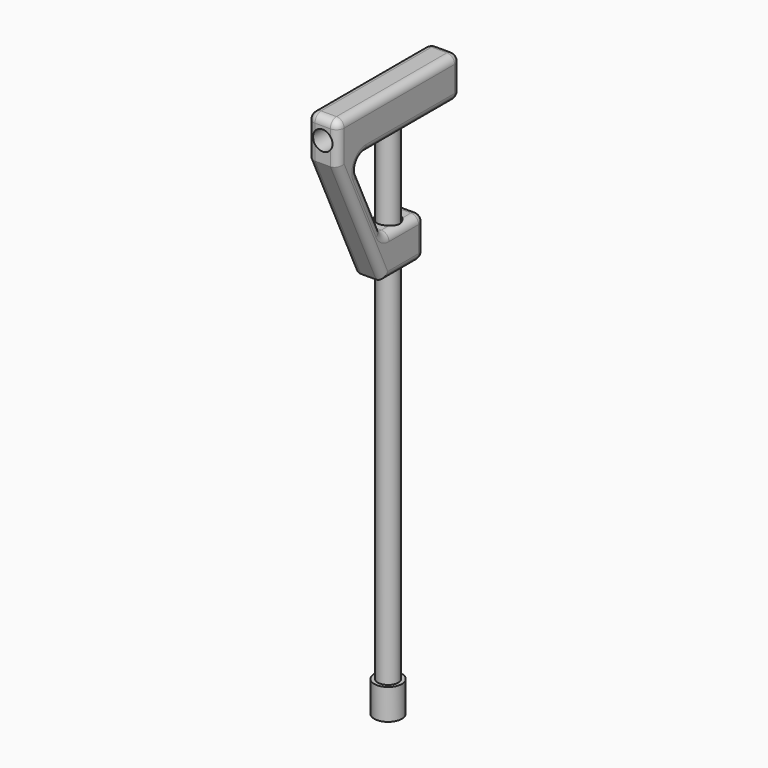
from build123d import *

# Parameters (mm, degrees)
F0_R          = 1.35
F1_DEPTH      = 3
F2_R          = 1
F3_DEPTH      = 50
F4_W          = 5
F4_H          = 4
F5_DEPTH      = 1.5
F6_R          = 1.1
F7_DEPTH      = 14.4
F8_R          = 0.95
F9_DEPTH      = 25
F10_R         = 1
F11_T1_DEPTH  = 2.5
F11_T3_DEPTH  = 2.5
F11_T5_DEPTH  = 13.5
F11_T7_DEPTH  = 10.8131369762
F11_T9_DEPTH  = 5.125
F11_T11_DEPTH = 1.5
F11_T13_DEPTH = 16.9923562858
F11_T15_DEPTH = 6.125
F11_T17_DEPTH = 3.6131369762
F11_T19_DEPTH = 6.6211781429
F11_S23_W     = 0.75
F11_S23_H     = 0.75
F11_T24_DEPTH = 0.75
F11_S29_W     = 0.75
F11_S29_H     = 0.75
F11_T30_DEPTH = 0.75
F11_S35_W     = 0.75
F11_S35_H     = 0.75
F11_T36_DEPTH = 0.75
F11_S41_W     = 0.75
F11_S41_H     = 0.75
F11_T42_DEPTH = 0.75
F11_S47_W     = 0.75
F11_S47_H     = 0.75
F11_T48_DEPTH = 0.75
F11_S53_W     = 0.75
F11_S53_H     = 0.75
F11_T54_DEPTH = 0.75
F11_S59_W     = 0.75
F11_S59_H     = 0.75
F11_T60_DEPTH = 0.75
F11_S65_W     = 0.75
F11_S65_H     = 0.75
F11_T66_DEPTH = 0.75
F11_S71_W     = 0.75
F11_S71_H     = 0.75
F11_T72_DEPTH = 0.75
F11_S77_W     = 0.75
F11_S77_H     = 0.75
F11_T78_DEPTH = 0.75
F11_T82_ANGLE = 64.9831065219
F11_T84_ANGLE = 115.0168934781
F11_T86_ANGLE = 64.9831065219
F11_T88_ANGLE = 115.0168934781


# Not quite as in the source:
# - a fillet or chamfer that OpenCascade refuses, or shapes differently, is made with other operations: its cross-section is extruded or revolved along the edge and cut away or added


with BuildPart() as f1:
    # F0 (on Top) → F1 (new body)
    with BuildSketch(Plane.XY):
        Circle(F0_R)
    extrude(amount=F1_DEPTH)

    # F2 (on face) → F3 (join)
    with BuildSketch(Plane.XY.offset(3)):
        Circle(F2_R)
    extrude(amount=F3_DEPTH)


with BuildPart() as f5:
    # F4 (on Right) → F5 (new body, symmetric)
    with BuildSketch(Plane.YZ):
        Polygon((7, 50.6), (7, 54.6), (-8, 54.6), (-8, 50.6), (-6.1333333333, 50.6), align=None)
        with Locations((0.1, 40.6)):
            Rectangle(F4_W, F4_H)
        Polygon((-6.1333333333, 50.6), (-8, 50.6), (-2.4, 38.6), (-2.4, 42.6), align=None)
    extrude(amount=F5_DEPTH, both=True)

    # F6 (on face) → F7 (cut, through all)
    with BuildSketch(Plane(origin=(0, 0, 38.6), x_dir=(1, 0, 0), z_dir=(0, 0, -1))):
        Circle(F6_R)
    extrude(amount=-F7_DEPTH, mode=Mode.SUBTRACT)

    # F8 (on face) → F9 (cut)
    with BuildSketch(Plane(origin=(0, 7, 0), x_dir=(-1, 0, 0), z_dir=(0, 1, 0))):
        with Locations((0, 52.6)):
            Circle(F8_R)
    extrude(amount=-F9_DEPTH, mode=Mode.SUBTRACT)

    # F10
    f10_edges = [f5.edges().sort_by_distance(p)[0] for p in [
        (0, -6.133333, 50.6),
        (0, -2.4, 42.6),
    ]]
    fillet(f10_edges, radius=F10_R)

    # F11: fillet of radius 0.75 on 27 edges, made by hand

    # F11_s2 → F11_t1 (cut)
    with BuildSketch(Plane.XY.offset(39.35)):
        with BuildLine():
            ThreePointArc((-1.5, 1.85), (-1.2803300859, 2.3803300859), (-0.75, 2.6))
            Line((-0.75, 2.6), (-1.5, 2.6))
            Line((-1.5, 2.6), (-1.5, 1.85))
        make_face()
        with BuildLine():
            ThreePointArc((0.75, 2.6), (1.2803300859, 2.3803300859), (1.5, 1.85))
            Line((1.5, 1.85), (1.5, 2.6))
            Line((1.5, 2.6), (0.75, 2.6))
        make_face()
    extrude(amount=F11_T1_DEPTH, mode=Mode.SUBTRACT)

    # F11_s4 → F11_t3 (cut)
    with BuildSketch(Plane.XY.offset(51.35)):
        with BuildLine():
            ThreePointArc((-1.5, 6.25), (-1.2803300859, 6.7803300859), (-0.75, 7))
            Line((-0.75, 7), (-1.5, 7))
            Line((-1.5, 7), (-1.5, 6.25))
        make_face()
        with BuildLine():
            ThreePointArc((0.75, 7), (1.2803300859, 6.7803300859), (1.5, 6.25))
            Line((1.5, 6.25), (1.5, 7))
            Line((1.5, 7), (0.75, 7))
        make_face()
    extrude(amount=F11_T3_DEPTH, mode=Mode.SUBTRACT)

    # F11_s6 → F11_t5 (cut)
    with BuildSketch(Plane.XZ.offset(-6.25)):
        with BuildLine():
            ThreePointArc((-1.5, 53.85), (-1.2803300859, 54.3803300859), (-0.75, 54.6))
            Line((-0.75, 54.6), (-1.5, 54.6))
            Line((-1.5, 54.6), (-1.5, 53.85))
        make_face()
        with BuildLine():
            ThreePointArc((0.75, 54.6), (1.2803300859, 54.3803300859), (1.5, 53.85))
            Line((1.5, 53.85), (1.5, 54.6))
            Line((1.5, 54.6), (0.75, 54.6))
        make_face()
    extrude(amount=F11_T5_DEPTH, mode=Mode.SUBTRACT)

    # F11_s8 → F11_t7 (cut)
    with BuildSketch(Plane.XZ.offset(-6.25)):
        with BuildLine():
            ThreePointArc((-1.5, 51.35), (-1.2803300859, 50.8196699141), (-0.75, 50.6))
            Line((-0.75, 50.6), (-1.5, 50.6))
            Line((-1.5, 50.6), (-1.5, 51.35))
        make_face()
        with BuildLine():
            ThreePointArc((0.75, 50.6), (1.2803300859, 50.8196699141), (1.5, 51.35))
            Line((1.5, 51.35), (1.5, 50.6))
            Line((1.5, 50.6), (0.75, 50.6))
        make_face()
    extrude(amount=F11_T7_DEPTH, mode=Mode.SUBTRACT)

    # F11_s10 → F11_t9 (cut)
    with BuildSketch(Plane.XY.offset(48.725)):
        with BuildLine():
            ThreePointArc((-1.5, -7.25), (-1.2803300859, -7.7803300859), (-0.75, -8))
            Line((-0.75, -8), (-1.5, -8))
            Line((-1.5, -8), (-1.5, -7.25))
        make_face()
        with BuildLine():
            ThreePointArc((0.75, -8), (1.2803300859, -7.7803300859), (1.5, -7.25))
            Line((1.5, -7.25), (1.5, -8))
            Line((1.5, -8), (0.75, -8))
        make_face()
    extrude(amount=F11_T9_DEPTH, mode=Mode.SUBTRACT)

    # F11_s12 → F11_t11 (cut)
    with BuildSketch(Plane.YZ.offset(-0.75)):
        with BuildLine():
            ThreePointArc((-8, 53.85), (-7.7803300859, 54.3803300859), (-7.25, 54.6))
            Line((-7.25, 54.6), (-8, 54.6))
            Line((-8, 54.6), (-8, 53.85))
        make_face()
        with BuildLine():
            ThreePointArc((7, 53.85), (6.7803300859, 54.3803300859), (6.25, 54.6))
            Line((6.25, 54.6), (7, 54.6))
            Line((7, 54.6), (7, 53.85))
        make_face()
        with BuildLine():
            ThreePointArc((6.25, 50.6), (6.7803300859, 50.8196699141), (7, 51.35))
            Line((7, 51.35), (7, 50.6))
            Line((7, 50.6), (6.25, 50.6))
        make_face()
        with BuildLine():
            ThreePointArc((2.6, 39.35), (2.3803300859, 38.8196699141), (1.85, 38.6))
            Line((1.85, 38.6), (2.6, 38.6))
            Line((2.6, 38.6), (2.6, 39.35))
        make_face()
        with BuildLine():
            ThreePointArc((1.85, 42.6), (2.3803300859, 42.3803300859), (2.6, 41.85))
            Line((2.6, 41.85), (2.6, 42.6))
            Line((2.6, 42.6), (1.85, 42.6))
        make_face()
    extrude(amount=F11_T11_DEPTH, mode=Mode.SUBTRACT)

    # F11_s14 → F11_t13 (cut)
    with BuildSketch(Plane(origin=(0, -21.6140781307, 46.3158817087), x_dir=(1, 0, 0), z_dir=(0, 0.4228854653, -0.90618314))):
        with BuildLine():
            ThreePointArc((-1.5, -14.8985394258), (-1.2803300859, -14.3682093399), (-0.75, -14.1485394258))
            Line((-0.75, -14.1485394258), (-1.5, -14.1485394258))
            Line((-1.5, -14.1485394258), (-1.5, -14.8985394258))
        make_face()
        with BuildLine():
            ThreePointArc((0.75, -14.1485394258), (1.2803300859, -14.3682093399), (1.5, -14.8985394258))
            Line((1.5, -14.8985394258), (1.5, -14.1485394258))
            Line((1.5, -14.1485394258), (0.75, -14.1485394258))
        make_face()
    extrude(amount=F11_T13_DEPTH, mode=Mode.SUBTRACT)

    # F11_s16 → F11_t15 (cut)
    with BuildSketch(Plane.XZ.offset(-1.85)):
        with BuildLine():
            ThreePointArc((-1.5, 39.35), (-1.2803300859, 38.8196699141), (-0.75, 38.6))
            Line((-0.75, 38.6), (-1.5, 38.6))
            Line((-1.5, 38.6), (-1.5, 39.35))
        make_face()
        with BuildLine():
            ThreePointArc((0.75, 38.6), (1.2803300859, 38.8196699141), (1.5, 39.35))
            Line((1.5, 39.35), (1.5, 38.6))
            Line((1.5, 38.6), (0.75, 38.6))
        make_face()
    extrude(amount=F11_T15_DEPTH, mode=Mode.SUBTRACT)

    # F11_s18 → F11_t17 (cut)
    with BuildSketch(Plane.XZ.offset(-1.85)):
        with BuildLine():
            ThreePointArc((-1.5, 41.85), (-1.2803300859, 42.3803300859), (-0.75, 42.6))
            Line((-0.75, 42.6), (-1.5, 42.6))
            Line((-1.5, 42.6), (-1.5, 41.85))
        make_face()
        with BuildLine():
            ThreePointArc((0.75, 42.6), (1.2803300859, 42.3803300859), (1.5, 41.85))
            Line((1.5, 41.85), (1.5, 42.6))
            Line((1.5, 42.6), (0.75, 42.6))
        make_face()
    extrude(amount=F11_T17_DEPTH, mode=Mode.SUBTRACT)

    # F11_s20 → F11_t19 (cut)
    with BuildSketch(Plane(origin=(0, -17.0233347147, 36.4785743887), x_dir=(1, 0, 0), z_dir=(0, -0.4228854653, 0.90618314))):
        with BuildLine():
            ThreePointArc((-1.5, 15.0900812871), (-1.2803300859, 15.620411373), (-0.75, 15.8400812871))
            Line((-0.75, 15.8400812871), (-1.5, 15.8400812871))
            Line((-1.5, 15.8400812871), (-1.5, 15.0900812871))
        make_face()
        with BuildLine():
            ThreePointArc((0.75, 15.8400812871), (1.2803300859, 15.620411373), (1.5, 15.0900812871))
            Line((1.5, 15.0900812871), (1.5, 15.8400812871))
            Line((1.5, 15.8400812871), (0.75, 15.8400812871))
        make_face()
    extrude(amount=F11_T19_DEPTH, mode=Mode.SUBTRACT)


with BuildPart() as f11_tool22:
    # F11_s23 → F11_t24 (new body)
    with BuildSketch(Plane.YZ.offset(-0.75)):
        with Locations((2.225, 38.975)):
            Rectangle(F11_S23_W, F11_S23_H)
    extrude(amount=-F11_T24_DEPTH)

    # F11_s25 → F11_t26 (revolve, cut)
    with BuildSketch(Plane(origin=(-0.75, 1.85, 39.35), x_dir=(0, -0.7071067812, 0.7071067812), z_dir=(0, -0.7071067812, -0.7071067812))):
        with BuildLine():
            ThreePointArc((0, -0.75), (0.75, 0), (0, 0.75))
            Line((0, 0.75), (0, -0.75))
        make_face()
    revolve(axis=Axis((-0.75, 1.85, 39.35), (-1, 0, 0)), mode=Mode.SUBTRACT)


with BuildPart() as f5_1:
    add(f5.part)

    # F11_t21: cut F11_tool22
    add(f11_tool22.part, mode=Mode.SUBTRACT)


with BuildPart() as f11_tool28:
    # F11_s29 → F11_t30 (new body)
    with BuildSketch(Plane.YZ.offset(-0.75)):
        with Locations((2.225, 42.225)):
            Rectangle(F11_S29_W, F11_S29_H)
    extrude(amount=-F11_T30_DEPTH)

    # F11_s31 → F11_t32 (revolve, cut)
    with BuildSketch(Plane(origin=(-0.75, 1.85, 41.85), x_dir=(0, -0.7071067812, -0.7071067812), z_dir=(0, 0.7071067812, -0.7071067812))):
        with BuildLine():
            ThreePointArc((0, -0.75), (0.75, 0), (0, 0.75))
            Line((0, 0.75), (0, -0.75))
        make_face()
    revolve(axis=Axis((-0.75, 1.85, 41.85), (-1, 0, 0)), mode=Mode.SUBTRACT)


with BuildPart() as f5_2:
    add(f5_1.part)

    # F11_t27: cut F11_tool28
    add(f11_tool28.part, mode=Mode.SUBTRACT)


with BuildPart() as f11_tool34:
    # F11_s35 → F11_t36 (new body)
    with BuildSketch(Plane.YZ.offset(-0.75)):
        with Locations((6.625, 50.975)):
            Rectangle(F11_S35_W, F11_S35_H)
    extrude(amount=-F11_T36_DEPTH)

    # F11_s37 → F11_t38 (revolve, cut)
    with BuildSketch(Plane(origin=(-0.75, 6.25, 51.35), x_dir=(0, -0.7071067812, 0.7071067812), z_dir=(0, -0.7071067812, -0.7071067812))):
        with BuildLine():
            ThreePointArc((0, -0.75), (0.75, 0), (0, 0.75))
            Line((0, 0.75), (0, -0.75))
        make_face()
    revolve(axis=Axis((-0.75, 6.25, 51.35), (-1, 0, 0)), mode=Mode.SUBTRACT)


with BuildPart() as f5_3:
    add(f5_2.part)

    # F11_t33: cut F11_tool34
    add(f11_tool34.part, mode=Mode.SUBTRACT)


with BuildPart() as f11_tool40:
    # F11_s41 → F11_t42 (new body)
    with BuildSketch(Plane.YZ.offset(-0.75)):
        with Locations((6.625, 54.225)):
            Rectangle(F11_S41_W, F11_S41_H)
    extrude(amount=-F11_T42_DEPTH)

    # F11_s43 → F11_t44 (revolve, cut)
    with BuildSketch(Plane(origin=(-0.75, 6.25, 53.85), x_dir=(0, -0.7071067812, -0.7071067812), z_dir=(0, 0.7071067812, -0.7071067812))):
        with BuildLine():
            ThreePointArc((0, -0.75), (0.75, 0), (0, 0.75))
            Line((0, 0.75), (0, -0.75))
        make_face()
    revolve(axis=Axis((-0.75, 6.25, 53.85), (-1, 0, 0)), mode=Mode.SUBTRACT)


with BuildPart() as f5_4:
    add(f5_3.part)

    # F11_t39: cut F11_tool40
    add(f11_tool40.part, mode=Mode.SUBTRACT)


with BuildPart() as f11_tool46:
    # F11_s47 → F11_t48 (new body)
    with BuildSketch(Plane.XY.offset(51.35)):
        with Locations((1.125, 6.625)):
            Rectangle(F11_S47_W, F11_S47_H)
    extrude(amount=-F11_T48_DEPTH)

    # F11_s49 → F11_t50 (revolve, cut)
    with BuildSketch(Plane(origin=(0.75, 6.25, 51.35), x_dir=(-0.7071067812, -0.7071067812, 0), z_dir=(0.7071067812, -0.7071067812, 0))):
        with BuildLine():
            ThreePointArc((0, -0.75), (0.75, 0), (0, 0.75))
            Line((0, 0.75), (0, -0.75))
        make_face()
    revolve(axis=Axis((0.75, 6.25, 51.35), (0, 0, -1)), mode=Mode.SUBTRACT)


with BuildPart() as f5_5:
    add(f5_4.part)

    # F11_t45: cut F11_tool46
    add(f11_tool46.part, mode=Mode.SUBTRACT)


with BuildPart() as f11_tool52:
    # F11_s53 → F11_t54 (new body)
    with BuildSketch(Plane.XZ.offset(-6.25)):
        with Locations((1.125, 54.225)):
            Rectangle(F11_S53_W, F11_S53_H)
    extrude(amount=-F11_T54_DEPTH)

    # F11_s55 → F11_t56 (revolve, cut)
    with BuildSketch(Plane(origin=(0.75, 6.25, 53.85), x_dir=(-0.7071067812, 0, -0.7071067812), z_dir=(0.7071067812, 0, -0.7071067812))):
        with BuildLine():
            ThreePointArc((0, -0.75), (0.75, 0), (0, 0.75))
            Line((0, 0.75), (0, -0.75))
        make_face()
    revolve(axis=Axis((0.75, 6.25, 53.85), (0, 1, 0)), mode=Mode.SUBTRACT)


with BuildPart() as f5_6:
    add(f5_5.part)

    # F11_t51: cut F11_tool52
    add(f11_tool52.part, mode=Mode.SUBTRACT)


with BuildPart() as f11_tool58:
    # F11_s59 → F11_t60 (new body)
    with BuildSketch(Plane.XZ.offset(-1.85)):
        with Locations((1.125, 38.975)):
            Rectangle(F11_S59_W, F11_S59_H)
    extrude(amount=-F11_T60_DEPTH)

    # F11_s61 → F11_t62 (revolve, cut)
    with BuildSketch(Plane(origin=(0.75, 1.85, 39.35), x_dir=(-0.7071067812, 0, 0.7071067812), z_dir=(-0.7071067812, 0, -0.7071067812))):
        with BuildLine():
            ThreePointArc((0, -0.75), (0.75, 0), (0, 0.75))
            Line((0, 0.75), (0, -0.75))
        make_face()
    revolve(axis=Axis((0.75, 1.85, 39.35), (0, 1, 0)), mode=Mode.SUBTRACT)


with BuildPart() as f5_7:
    add(f5_6.part)

    # F11_t57: cut F11_tool58
    add(f11_tool58.part, mode=Mode.SUBTRACT)


with BuildPart() as f11_tool64:
    # F11_s65 → F11_t66 (new body)
    with BuildSketch(Plane.XY.offset(41.85)):
        with Locations((1.125, 2.225)):
            Rectangle(F11_S65_W, F11_S65_H)
    extrude(amount=F11_T66_DEPTH)

    # F11_s67 → F11_t68 (revolve, cut)
    with BuildSketch(Plane(origin=(0.75, 1.85, 41.85), x_dir=(-0.7071067812, -0.7071067812, 0), z_dir=(-0.7071067812, 0.7071067812, 0))):
        with BuildLine():
            ThreePointArc((0, -0.75), (0.75, 0), (0, 0.75))
            Line((0, 0.75), (0, -0.75))
        make_face()
    revolve(axis=Axis((0.75, 1.85, 41.85), (0, 0, 1)), mode=Mode.SUBTRACT)


with BuildPart() as f5_8:
    add(f5_7.part)

    # F11_t63: cut F11_tool64
    add(f11_tool64.part, mode=Mode.SUBTRACT)


with BuildPart() as f11_tool70:
    # F11_s71 → F11_t72 (new body)
    with BuildSketch(Plane.YZ.offset(-0.75)):
        with Locations((-7.625, 54.225)):
            Rectangle(F11_S71_W, F11_S71_H)
    extrude(amount=-F11_T72_DEPTH)

    # F11_s73 → F11_t74 (revolve, cut)
    with BuildSketch(Plane(origin=(-0.75, -7.25, 53.85), x_dir=(0, 0.7071067812, -0.7071067812), z_dir=(0, 0.7071067812, 0.7071067812))):
        with BuildLine():
            ThreePointArc((0, -0.75), (0.75, 0), (0, 0.75))
            Line((0, 0.75), (0, -0.75))
        make_face()
    revolve(axis=Axis((-0.75, -7.25, 53.85), (-1, 0, 0)), mode=Mode.SUBTRACT)


with BuildPart() as f5_9:
    add(f5_8.part)

    # F11_t69: cut F11_tool70
    add(f11_tool70.part, mode=Mode.SUBTRACT)


with BuildPart() as f11_tool76:
    # F11_s77 → F11_t78 (new body)
    with BuildSketch(Plane.XZ.offset(7.25)):
        with Locations((1.125, 54.225)):
            Rectangle(F11_S77_W, F11_S77_H)
    extrude(amount=F11_T78_DEPTH)

    # F11_s79 → F11_t80 (revolve, cut)
    with BuildSketch(Plane(origin=(0.75, -7.25, 53.85), x_dir=(-0.7071067812, 0, -0.7071067812), z_dir=(-0.7071067812, 0, 0.7071067812))):
        with BuildLine():
            ThreePointArc((0, -0.75), (0.75, 0), (0, 0.75))
            Line((0, 0.75), (0, -0.75))
        make_face()
    revolve(axis=Axis((0.75, -7.25, 53.85), (0, -1, 0)), mode=Mode.SUBTRACT)


with BuildPart() as f5_10:
    add(f5_9.part)

    # F11_t75: cut F11_tool76
    add(f11_tool76.part, mode=Mode.SUBTRACT)

    # F11_s81 → F11_t82 (revolve, cut)
    with BuildSketch(Plane.XZ.offset(1.7631369762)):
        with BuildLine():
            ThreePointArc((-1.5, 41.85), (-1.2803300859, 42.3803300859), (-0.75, 42.6))
            Line((-0.75, 42.6), (-1.5, 42.6))
            Line((-1.5, 42.6), (-1.5, 41.85))
        make_face()
    revolve(axis=Axis((-1.5, -1.7631369762, 43.6), (-1, 0, 0)), revolution_arc=F11_T82_ANGLE, mode=Mode.SUBTRACT)

    # F11_s83 → F11_t84 (revolve, cut)
    with BuildSketch(Plane.XZ.offset(4.5631369762)):
        with BuildLine():
            ThreePointArc((-1.5, 51.35), (-1.2803300859, 50.8196699141), (-0.75, 50.6))
            Line((-0.75, 50.6), (-1.5, 50.6))
            Line((-1.5, 50.6), (-1.5, 51.35))
        make_face()
    revolve(axis=Axis((-1.5, -4.5631369762, 49.6), (1, 0, 0)), revolution_arc=F11_T84_ANGLE, mode=Mode.SUBTRACT)

    # F11_s85 → F11_t86 (revolve, cut)
    with BuildSketch(Plane.XZ.offset(1.7631369762)):
        with BuildLine():
            ThreePointArc((0.75, 42.6), (1.2803300859, 42.3803300859), (1.5, 41.85))
            Line((1.5, 41.85), (1.5, 42.6))
            Line((1.5, 42.6), (0.75, 42.6))
        make_face()
    revolve(axis=Axis((1.5, -1.7631369762, 43.6), (-1, 0, 0)), revolution_arc=F11_T86_ANGLE, mode=Mode.SUBTRACT)

    # F11_s87 → F11_t88 (revolve, cut)
    with BuildSketch(Plane.XZ.offset(4.5631369762)):
        with BuildLine():
            ThreePointArc((0.75, 50.6), (1.2803300859, 50.8196699141), (1.5, 51.35))
            Line((1.5, 51.35), (1.5, 50.6))
            Line((1.5, 50.6), (0.75, 50.6))
        make_face()
    revolve(axis=Axis((1.5, -4.5631369762, 49.6), (1, 0, 0)), revolution_arc=F11_T88_ANGLE, mode=Mode.SUBTRACT)


solid = Compound([f1.part, f5_10.part])
